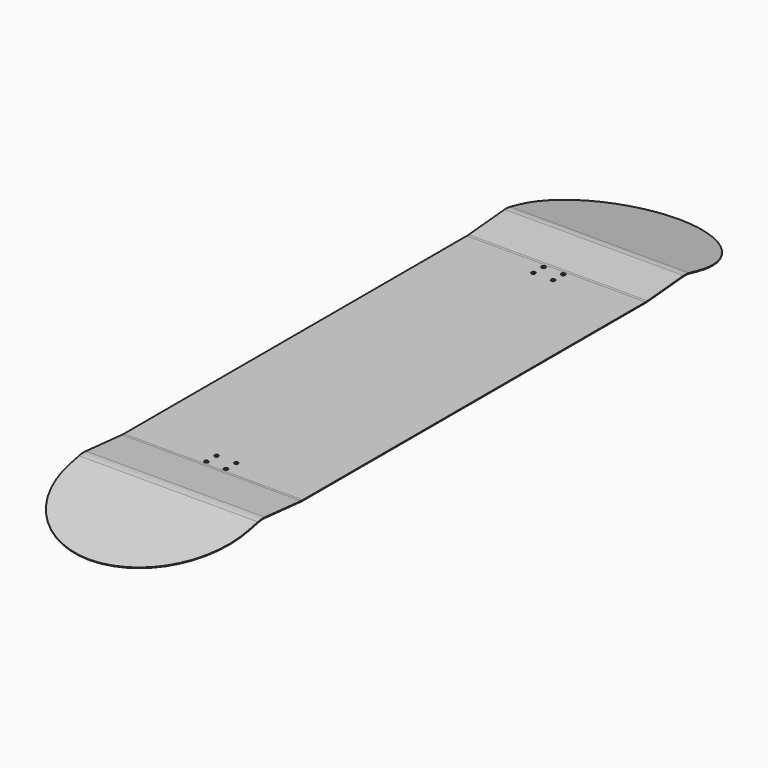
from build123d import *

# Parameters (mm, degrees)
F0_W        = 201.6125
F0_H        = 482.6
F1_DEPTH    = 0.79375
F3_DEPTH    = 201.6125
F4_T1_DEPTH = 508.79375
F4_T3_DEPTH = 508.79375
F5_R        = 2.15265
F6_DEPTH    = 0.79375


# Not quite as in the source:
# - a fillet or chamfer that OpenCascade refuses, or shapes differently, is made with other operations: its cross-section is extruded or revolved along the edge and cut away or added


with BuildPart() as f1:
    # F0 (on Top) → F1 (new body)
    with BuildSketch(Plane.XY):
        Rectangle(F0_W, F0_H)
    extrude(amount=F1_DEPTH)

    # F2 (on face) → F3 (join, through all)
    with BuildSketch(Plane.YZ.offset(100.80625)):
        with BuildLine():
            ThreePointArc((244.0671948322, 0.9145683356), (242.6849155488, 0.8239689648), (241.3, 0.79375))
            Line((241.3, 0.79375), (241.3, 0))
            ThreePointArc((241.3, 0), (242.7195384376, 0.0309744389), (244.136374703, 0.123838794))
            Line((244.136374703, 0.123838794), (294.7430653661, 4.5513505256))
            ThreePointArc((294.7430653661, 4.5513505256), (298.5031396949, 4.5918955138), (302.2254864388, 4.0590375853))
            Line((302.2254864388, 4.0590375853), (413.8036674178, -20.7361137434))
            Line((413.8036674178, -20.7361137434), (413.9758559687, -19.9612652644))
            Line((413.9758559687, -19.9612652644), (302.3976749897, 4.8338860643))
            ThreePointArc((302.3976749897, 4.8338860643), (298.5552525443, 5.3839329582), (294.6738854953, 5.3420800672))
            Line((294.6738854953, 5.3420800672), (244.0671948322, 0.9145683356))
        make_face()
        with BuildLine():
            Line((-241.3, 0), (-241.3, 0.79375))
            ThreePointArc((-241.3, 0.79375), (-242.6849155488, 0.8239689648), (-244.0671948322, 0.9145683356))
            Line((-244.0671948322, 0.9145683356), (-294.6738854953, 5.3420800672))
            ThreePointArc((-294.6738854953, 5.3420800672), (-299.6272962644, 5.3969871417), (-304.5316552149, 4.699451251))
            Line((-304.5316552149, 4.699451251), (-416.1396714134, -19.9610580753))
            Line((-416.1396714134, -19.9610580753), (-415.9684178764, -20.7361137434))
            Line((-415.9684178764, -20.7361137434), (-304.3604016779, 3.924395583))
            ThreePointArc((-304.3604016779, 3.924395583), (-299.5756612384, 4.6049184032), (-294.7430653661, 4.5513505256))
            Line((-294.7430653661, 4.5513505256), (-244.136374703, 0.123838794))
            ThreePointArc((-244.136374703, 0.123838794), (-242.7195384376, 0.0309744389), (-241.3, 0))
        make_face()
    extrude(amount=-F3_DEPTH)

    # F4: fillet of radius 101.6 on 4 edges, made by hand

    # F4_s2 → F4_t1 (cut)
    with BuildSketch(Plane(origin=(0, -40.0183995531, -180.082797989), x_dir=(1, 0, 0), z_dir=(0, 0.2169304578, 0.9761870602))):
        with BuildLine():
            ThreePointArc((100.80625, 306.8480802377), (71.0482989686, 378.6901292062), (-0.79375, 408.4480802377))
            Line((-0.79375, 408.4480802377), (100.80625, 408.4480802377))
            Line((100.80625, 408.4480802377), (100.80625, 306.8480802377))
        make_face()
        with BuildLine():
            ThreePointArc((0.79375, 408.4480802377), (-71.0482989686, 378.6901292062), (-100.80625, 306.8480802377))
            Line((-100.80625, 306.8480802377), (-100.80625, 408.4480802377))
            Line((-100.80625, 408.4480802377), (0.79375, 408.4480802377))
        make_face()
    extrude(amount=F4_T1_DEPTH, mode=Mode.SUBTRACT)

    # F4_s4 → F4_t3 (cut)
    with BuildSketch(Plane(origin=(0, -69.9668558158, 316.6545294712), x_dir=(1, 0, 0), z_dir=(0, 0.2157524875, -0.9764480857))):
        with BuildLine():
            ThreePointArc((100.80625, 309.0454334801), (71.0482989686, 380.8874824486), (-0.79375, 410.6454334801))
            Line((-0.79375, 410.6454334801), (100.80625, 410.6454334801))
            Line((100.80625, 410.6454334801), (100.80625, 309.0454334801))
        make_face()
        with BuildLine():
            ThreePointArc((0.79375, 410.6454334801), (-71.0482989686, 380.8874824486), (-100.80625, 309.0454334801))
            Line((-100.80625, 309.0454334801), (-100.80625, 410.6454334801))
            Line((-100.80625, 410.6454334801), (0.79375, 410.6454334801))
        make_face()
    extrude(amount=F4_T3_DEPTH, mode=Mode.SUBTRACT)

    # F5 (on face) → F6 (cut, through all)
    with BuildSketch(Plane.XY.offset(0.79375)):
        with Locations((-11.1125, 237.33125)):
            Circle(F5_R)
        with Locations((11.1125, 237.33125)):
            Circle(F5_R)
        with Locations((11.1125, 223.04375)):
            Circle(F5_R)
        with Locations((-11.1125, 223.04375)):
            Circle(F5_R)
        with Locations((11.1125, -223.04375)):
            Circle(F5_R)
        with Locations((-11.1125, -223.04375)):
            Circle(F5_R)
        with Locations((-11.1125, -237.33125)):
            Circle(F5_R)
        with Locations((11.1125, -237.33125)):
            Circle(F5_R)
    extrude(amount=-F6_DEPTH, mode=Mode.SUBTRACT)


solid = f1.part
